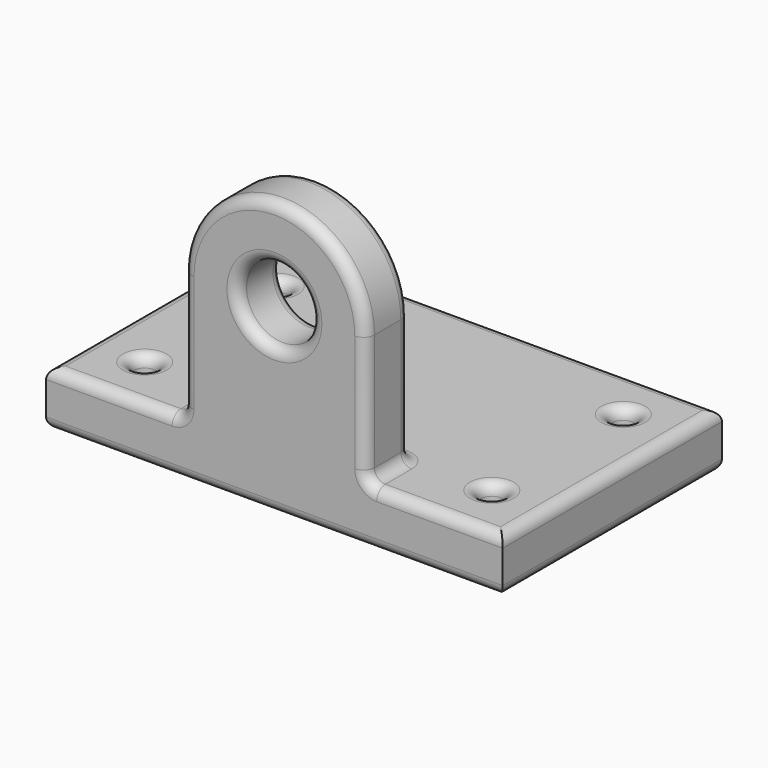
from build123d import *

# Parameters (mm, degrees)
F0_W     = 125
F0_H     = 75
F0_R     = 3
F1_DEPTH = 15
F2_W     = 50
F2_H     = 15
F3_DEPTH = 15
F4_R     = 3


with BuildPart() as f1:
    # F0 (on Top) → F1 (new body)
    with BuildSketch(Plane.XY):
        Rectangle(F0_W, F0_H)
        with Locations((-47.5, -22.5)):
            Circle(F0_R, mode=Mode.SUBTRACT)
        with Locations((47.5, -22.5)):
            Circle(F0_R, mode=Mode.SUBTRACT)
        with Locations((-47.5, 22.5)):
            Circle(F0_R, mode=Mode.SUBTRACT)
        with Locations((47.5, 22.5)):
            Circle(F0_R, mode=Mode.SUBTRACT)
    extrude(amount=F1_DEPTH)

    # F2 (on face) → F3 (join)
    with BuildSketch(Plane.XZ.offset(37.5)):
        with BuildLine():
            Line((10, 50), (25, 50))
            ThreePointArc((25, 50), (0, 75), (-25, 50))
            Line((-25, 50), (-10, 50))
            ThreePointArc((-10, 50), (0, 60), (10, 50))
        make_face()
        with BuildLine():
            ThreePointArc((-25, 50), (0, 25), (25, 50))
            Line((25, 50), (10, 50))
            ThreePointArc((10, 50), (0, 40), (-10, 50))
            Line((-10, 50), (-25, 50))
        make_face()
        with BuildLine():
            Line((25, 15), (25, 50))
            ThreePointArc((25, 50), (0, 25), (-25, 50))
            Line((-25, 50), (-25, 15))
            Line((-25, 15), (25, 15))
        make_face()
        with Locations((0, 7.5)):
            Rectangle(F2_W, F2_H)
    extrude(amount=-F3_DEPTH)

    # F4
    f4_edges = [f1.edges().sort_by_distance(p)[0] for p in [
        (43.75, -37.5, 15),
        (25, -30, 15),
        (0, -22.5, 15),
        (-25, -30, 15),
        (-43.75, -37.5, 15),
        (-62.5, 0, 15),
        (0, 37.5, 15),
        (62.5, 0, 15),
        (-50.5, -22.5, 15),
        (44.5, -22.5, 15),
        (-50.5, 22.5, 15),
        (44.5, 22.5, 15),
        (10, -30, 50),
        (-10, -37.5, 50),
        (-10, -22.5, 50),
        (25, -22.5, 32.5),
        (0, -22.5, 75),
        (62.5, 0, 0),
        (0, 37.5, 0),
        (-62.5, 0, 0),
        (0, -37.5, 0),
        (-50.5, -22.5, 0),
        (44.5, -22.5, 0),
        (-50.5, 22.5, 0),
        (44.5, 22.5, 0),
        (-25, -37.5, 32.5),
        (-25, -22.5, 32.5),
        (0, -37.5, 75),
        (25, -37.5, 32.5),
    ]]
    fillet(f4_edges, radius=F4_R)


solid = f1.part
